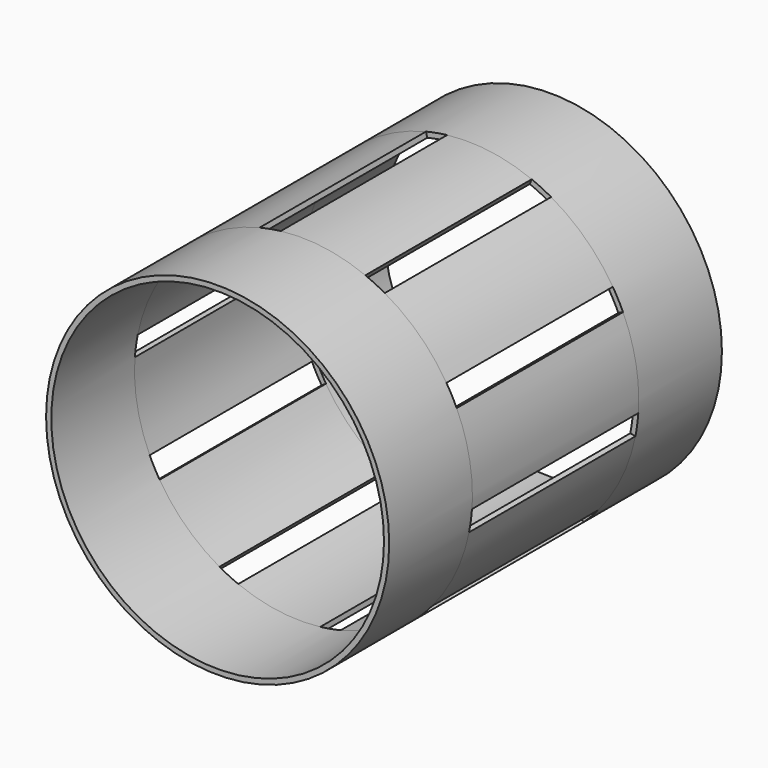
from build123d import *
from build123d import SkipClean  # not in build123d's __all__

# Parameters (mm, degrees)
F1_DEPTH = 20
F2_R     = 16.5
F2_R_2   = 16
F3_DEPTH = 10
F4_R     = 16.5
F4_R_2   = 16
F5_DEPTH = 10


with BuildPart() as f1:
    # F0 (on Front) → F1 (new body)
    with BuildSketch(Plane.XZ):
        with BuildLine():
            Line((-3.8441673982, 15.5313353262), (-3.9642976294, 16.0166895551))
            ThreePointArc((-3.9642976294, 16.0166895551), (-7.8229406478, 14.52761507), (-11.1900395345, 12.1257171011))
            Line((-11.1900395345, 12.1257171011), (-10.8509474274, 11.7582711284))
            ThreePointArc((-10.8509474274, 11.7582711284), (-7.5858818403, 14.0873843103), (-3.8441673982, 15.5313353262))
        make_face()
    extrude(amount=F1_DEPTH)



with BuildPart() as f1b:
    # F0 (on Front) → F1, piece 2 (new body)
    with BuildSketch(Plane.XZ):
        with BuildLine():
            ThreePointArc((-15.6899392355, 3.1346142961), (-14.4174640671, 6.9380638419), (-12.2390866075, 10.3055693202))
            Line((-12.2390866075, 10.3055693202), (-12.621558064, 10.6276183614))
            ThreePointArc((-12.621558064, 10.6276183614), (-14.8680098192, 7.154878337), (-16.1802498366, 3.2325709928))
            Line((-16.1802498366, 3.2325709928), (-15.6899392355, 3.1346142961))
        make_face()
    extrude(amount=F1_DEPTH)


with BuildPart() as f1c:
    # F0 (on Front) → F1, piece 3 (new body)
    with BuildSketch(Plane.XZ):
        with BuildLine():
            Line((-15.959090724, 1.1434261073), (-16.4578123091, 1.1791581731))
            ThreePointArc((-16.4578123091, 1.1791581731), (-16.2336959024, -2.952476477), (-14.9887120925, -6.8984425639))
            Line((-14.9887120925, -6.8984425639), (-14.5345086958, -6.6893988498))
            ThreePointArc((-14.5345086958, -6.6893988498), (-15.7417657236, -2.8630074928), (-15.959090724, 1.1434261073))
        make_face()
    extrude(amount=F1_DEPTH)


with BuildPart() as f1d:
    # F0 (on Front) → F1, piece 4 (new body)
    with BuildSketch(Plane.XZ):
        with BuildLine():
            Line((-13.581495765, -8.458307915), (-14.0059175077, -8.7226300373))
            ThreePointArc((-14.0059175077, -8.7226300373), (-11.3966659743, -11.9317226195), (-8.0713200038, -14.3911011877))
            Line((-8.0713200038, -14.3911011877), (-7.8267345492, -13.9550072124))
            ThreePointArc((-7.8267345492, -13.9550072124), (-11.05131246, -11.5701552674), (-13.581495765, -8.458307915))
        make_face()
    extrude(amount=F1_DEPTH)


with BuildPart() as f1e:
    # F0 (on Front) → F1, piece 5 (new body)
    with BuildSketch(Plane.XZ):
        with BuildLine():
            Line((-6.0159922312, -14.8259177616), (-6.2039919884, -15.2892276917))
            ThreePointArc((-6.2039919884, -15.2892276917), (-2.2068058623, -16.3517585564), (1.9290419923, -16.3868482934))
            Line((1.9290419923, -16.3868482934), (1.8705861743, -15.890277133))
            ThreePointArc((1.8705861743, -15.890277133), (-2.1399329573, -15.8562507213), (-6.0159922312, -14.8259177616))
        make_face()
    extrude(amount=F1_DEPTH)


with BuildPart() as f1f:
    # F0 (on Front) → F1, piece 6 (new body)
    with BuildSketch(Plane.XZ):
        with BuildLine():
            Line((6.0190930987, 14.8246591282), (6.2071897581, 15.287929726))
            ThreePointArc((6.2071897581, 15.287929726), (2.210225959, 16.3512966217), (-1.9256144656, 16.3872514147))
            Line((-1.9256144656, 16.3872514147), (-1.8672625121, 15.8906680385))
            ThreePointArc((-1.8672625121, 15.8906680385), (2.1432494148, 15.8558027847), (6.0190930987, 14.8246591282))
        make_face()
    extrude(amount=F1_DEPTH)


with BuildPart() as f1g:
    # F0 (on Front) → F1, piece 7 (new body)
    with BuildSketch(Plane.XZ):
        with BuildLine():
            ThreePointArc((14.0077416326, 8.7197003592), (11.3991613724, 11.929338624), (8.0743298799, 14.3894126701))
            Line((8.0743298799, 14.3894126701), (7.8296532169, 13.9533698619))
            ThreePointArc((7.8296532169, 13.9533698619), (11.0537322399, 11.5678435142), (13.5832646134, 8.455467015))
            Line((13.5832646134, 8.455467015), (14.0077416326, 8.7197003592))
        make_face()
    extrude(amount=F1_DEPTH)


with BuildPart() as f1h:
    # F0 (on Front) → F1, piece 8 (new body)
    with BuildSketch(Plane.XZ):
        with BuildLine():
            ThreePointArc((16.4580585827, -1.17571582), (16.2336959024, 2.952476477), (14.9901546477, 6.8953073636))
            Line((14.9901546477, 6.8953073636), (14.5359075371, 6.6863586557))
            ThreePointArc((14.5359075371, 6.6863586557), (15.7417657236, 2.8630074928), (15.9593295347, -1.1400880679))
            Line((15.9593295347, -1.1400880679), (16.4580585827, -1.17571582))
        make_face()
    extrude(amount=F1_DEPTH)


with BuildPart() as f1i:
    # F0 (on Front) → F1, piece 9 (new body)
    with BuildSketch(Plane.XZ):
        with BuildLine():
            ThreePointArc((3.9676476045, -16.0158600296), (7.8259790826, -14.5259785005), (11.192575513, -12.1233763195))
            Line((11.192575513, -12.1233763195), (10.8534065581, -11.7560012795))
            ThreePointArc((10.8534065581, -11.7560012795), (7.5888282013, -14.0857973339), (3.8474158589, -15.5305309377))
            Line((3.8474158589, -15.5305309377), (3.9676476045, -16.0158600296))
        make_face()
    extrude(amount=F1_DEPTH)


with BuildPart() as f1j:
    # F0 (on Front) → F1, piece 10 (new body)
    with BuildSketch(Plane.XZ):
        with BuildLine():
            ThreePointArc((12.6237806679, -10.6249781952), (14.8695060132, -7.1517683773), (16.1809256095, -3.22918665))
            Line((16.1809256095, -3.22918665), (15.6905945304, -3.1313325091))
            ThreePointArc((15.6905945304, -3.1313325091), (14.4189149219, -6.9350481235), (12.2412418598, -10.303009159))
            Line((12.2412418598, -10.303009159), (12.6237806679, -10.6249781952))
        make_face()
    extrude(amount=F1_DEPTH)


with BuildPart() as f1_1:
    add(f1.part, clean=False)

    add(f1b.part)  # F3 merges F1b

    add(f1c.part)  # F3 merges F1c

    add(f1d.part)  # F3 merges F1d

    add(f1e.part)  # F3 merges F1e

    add(f1f.part)  # F3 merges F1f

    add(f1g.part)  # F3 merges F1g

    add(f1h.part)  # F3 merges F1h

    add(f1i.part)  # F3 merges F1i

    add(f1j.part)  # F3 merges F1j
    # F2 (on face) → F3 (join)
    with BuildSketch(Plane.XZ):
        Circle(F2_R)
        Circle(F2_R_2, mode=Mode.SUBTRACT)
    extrude(amount=-F3_DEPTH)

    # F4 (on face) → F5 (join)
    with BuildSketch(Plane.XZ.offset(20)):
        Circle(F4_R)
        Circle(F4_R_2, mode=Mode.SUBTRACT)
    with SkipClean():  # cleaning this boolean's faces spoils the solid; the shape is the same uncleaned
        extrude(amount=F5_DEPTH)


solid = f1_1.part
